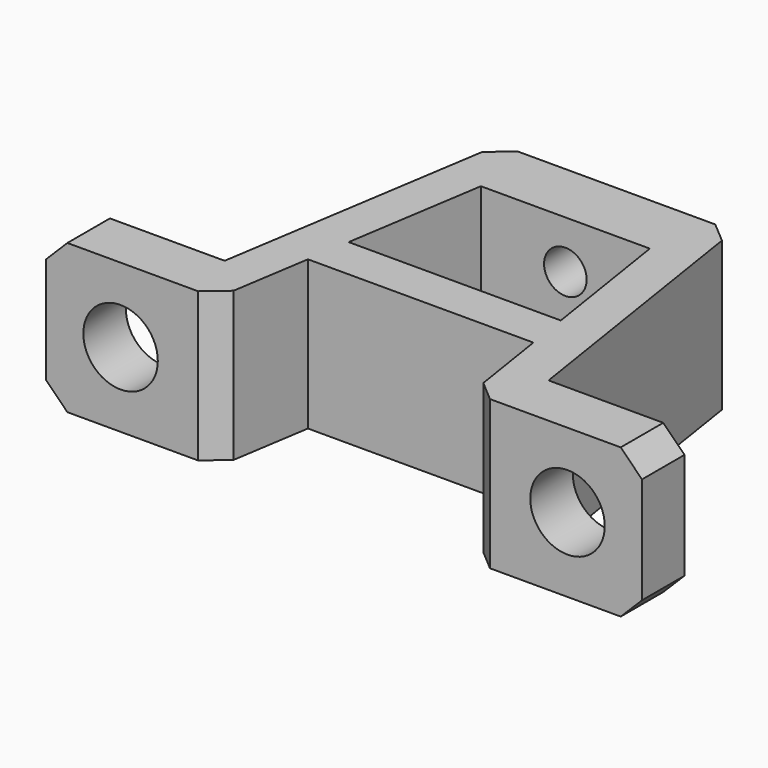
from build123d import *

# Parameters (mm, degrees)
F1_DEPTH    = 7
F2_R        = 1.75
F3_DEPTH    = 2.5
F4_R        = 1
F5_DEPTH    = 3
F6_T1_DEPTH = 7.6433659759
F6_T3_DEPTH = 11.4332708022


# Not quite as in the source:
# - a fillet or chamfer that OpenCascade refuses, or shapes differently, is made with other operations: its cross-section is extruded or revolved along the edge and cut away or added


with BuildPart() as f1:
    # F0 (on Top) → F1 (new body)
    with BuildSketch(Plane.XY):
        Polygon((0, 3), (0, 0), (1.53125, 0), (9.46875, 0), (11, 0), (11, 3), align=None)
        Polygon((1.53125, 0), (0, 0), (0, 3), (-2.109375, -10.5), (-2.5, -13), (-0.5, -13), (0.203125, -8.5), (0.515625, -6.5), align=None)
        Polygon((10.484375, -6.5), (0.515625, -6.5), (0.203125, -8.5), (10.796875, -8.5), align=None)
        Polygon((11, 0), (9.46875, 0), (10.484375, -6.5), (10.796875, -8.5), (11.5, -13), (13.5, -13), (13.109375, -10.5), (11, 3), align=None)
        Polygon((19.5, -10.5), (13.109375, -10.5), (13.5, -13), (19.5, -13), align=None)
        Polygon((-2.5, -13), (-2.109375, -10.5), (-8.5, -10.5), (-8.5, -13), align=None)
    extrude(amount=F1_DEPTH)

    # F2 (on face) → F3 (cut, through all)
    with BuildSketch(Plane.XZ.offset(13)):
        with Locations((-5, 3.5)):
            Circle(F2_R)
        with Locations((16, 3.5)):
            Circle(F2_R)
    extrude(amount=-F3_DEPTH, mode=Mode.SUBTRACT)

    # F4 (on face) → F5 (cut, through all)
    with BuildSketch(Plane(origin=(0, 3, 0), x_dir=(-1, 0, 0), z_dir=(0, 1, 0))):
        with Locations((-5.5, 4.75)):
            Circle(F4_R)
    extrude(amount=-F5_DEPTH, mode=Mode.SUBTRACT)

    # F6: chamfer of 1 on 8 edges, made by hand

    # F6_s2 → F6_t1 (cut)
    with BuildSketch(Plane.XZ.offset(7.928317012)):
        Polygon((-7.5, 7), (-8.5, 6), (-8.5, 7), align=None)
        Polygon((-7.5, 0), (-8.5, 1), (-8.5, 0), align=None)
        Polygon((18.5, 7), (19.5, 6), (19.5, 7), align=None)
        Polygon((18.5, 0), (19.5, 1), (19.5, 0), align=None)
    extrude(amount=F6_T1_DEPTH, mode=Mode.SUBTRACT)

    # F6_s4 → F6_t3 (cut)
    with BuildSketch(Plane.XY.offset(-2.2166354011)):
        Polygon((0.8558834213, 3), (-0.1321286125, 2.1543768803), (0, 3), align=None)
        Polygon((10.1441165787, 3), (11.1321286125, 2.1543768803), (11, 3), align=None)
        Polygon((-1.3558834213, -13), (-0.3678713875, -12.1543768803), (-0.5, -13), align=None)
        Polygon((11.3678713875, -12.1543768803), (12.3558834213, -13), (11.5, -13), align=None)
    extrude(amount=F6_T3_DEPTH, mode=Mode.SUBTRACT)


solid = f1.part
